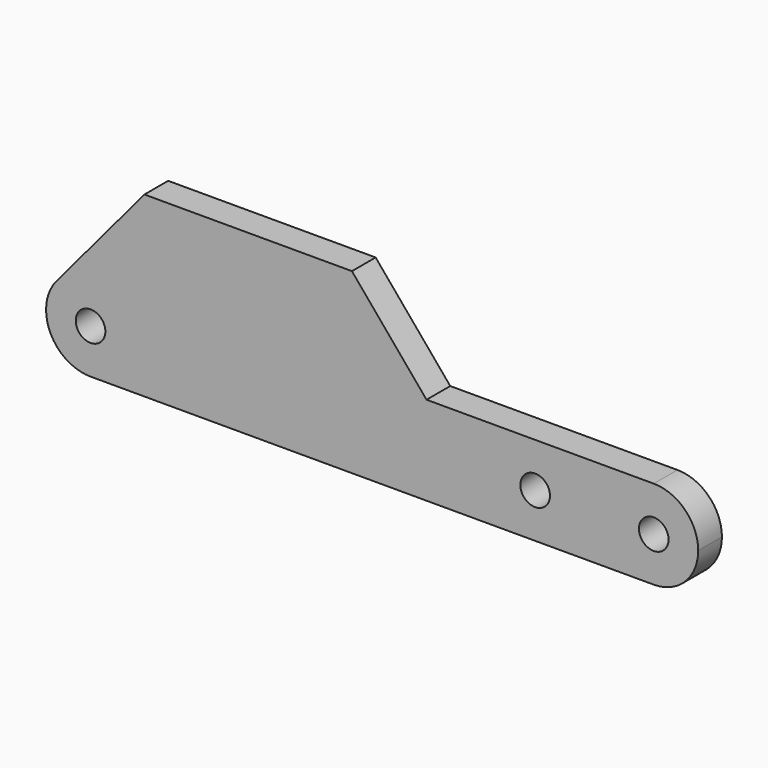
from build123d import *

# Parameters (mm, degrees)
F0_W      = 139.7
F0_H      = 19.05
F1_DEPTH  = 6.35
F2_R      = 3.175
F3_DEPTH  = 6.351
F4_R      = 3.175
F5_DEPTH  = 25.4
F6_R      = 9.52499
F7_R      = 9.52499
F8_R      = 3.175
F9_DEPTH  = 6.351
F11_DEPTH = 6.35


# Not quite as in the source:
# - a fillet or chamfer is up to 0.001 mm smaller than in the source, because OpenCascade refuses the exact size


with BuildPart() as f1:
    # F0 (on Front) → F1 (new body)
    with BuildSketch(Plane.XZ):
        with Locations((69.85, 9.525)):
            Rectangle(F0_W, F0_H)
    extrude(amount=F1_DEPTH)

    # F2 (on face) → F3 (cut, through all)
    with BuildSketch(Plane.XZ.offset(6.35)):
        with Locations((130.175, 9.525)):
            Circle(F2_R)
    extrude(amount=-F3_DEPTH, mode=Mode.SUBTRACT)

    # F4 (on face) → F5 (cut)
    with BuildSketch(Plane.XZ.offset(6.35)):
        with Locations((104.775, 9.525)):
            Circle(F4_R)
    extrude(amount=-F5_DEPTH, mode=Mode.SUBTRACT)

    # F6 (radius 9.525 in the source; OpenCascade refuses exactly that, so slightly less here)
    f6_edges = [f1.edges().sort_by_distance(p)[0] for p in [
        (139.7, -3.175, 19.05),
        (139.7, -3.175, 0),
    ]]
    fillet(f6_edges, radius=F6_R)

    # F7 (radius 9.525 in the source; OpenCascade refuses exactly that, so slightly less here)
    f7_edges = [f1.edges().sort_by_distance(p)[0] for p in [
        (0, -3.175, 19.05),
        (0, -3.175, 0),
    ]]
    fillet(f7_edges, radius=F7_R)

    # F8 (on face) → F9 (cut, through all)
    with BuildSketch(Plane.XZ.offset(6.35)):
        with Locations((9.525, 9.525)):
            Circle(F8_R)
    extrude(amount=-F9_DEPTH, mode=Mode.SUBTRACT)

    # F10 (on face) → F11 (join)
    with BuildSketch(Plane.XZ.offset(6.35)):
        with BuildLine():
            Line((21.06826753, 38.1), (2.2284266793, 15.6475519823))
            ThreePointArc((2.2284266793, 15.6475519823), (5.4995610569, 18.1575816715), (9.525, 19.05))
            Line((9.525, 19.05), (81.5031155039, 19.05))
            Line((81.5031155039, 19.05), (65.51826753, 38.1))
            Line((65.51826753, 38.1), (21.06826753, 38.1))
        make_face()
    extrude(amount=-F11_DEPTH)


solid = f1.part
